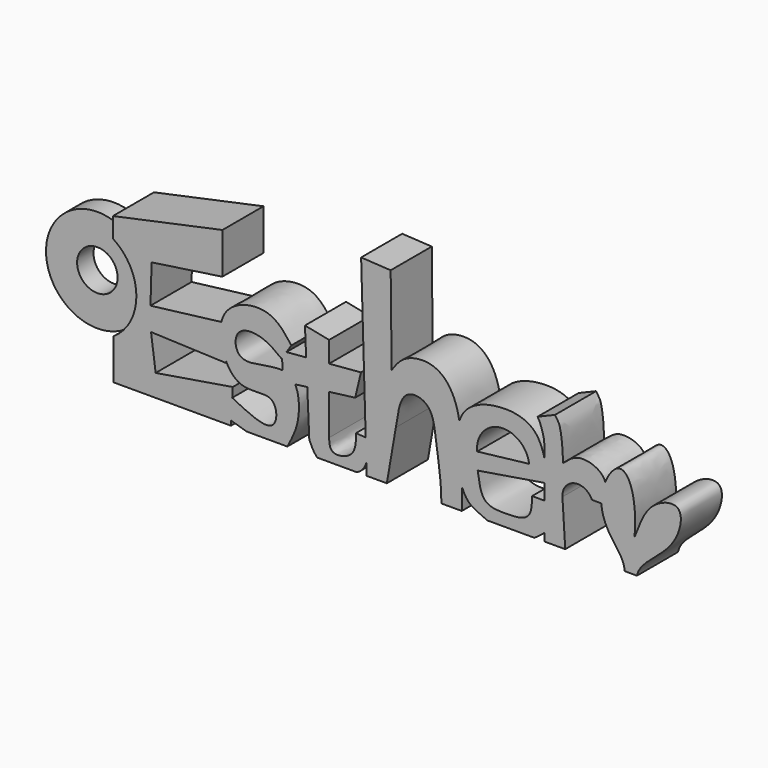
from build123d import *

# Parameters (mm, degrees)
F1_DEPTH = 5
F2_START = 1.5
F2_DEPTH = 2


# Not quite as in the source:
# - a feature names something its author has since deleted; it is built from what else it names


with BuildPart() as f1:
    # F0 (on Front) → F1 (new body)
    with BuildSketch(Plane.XZ):
        with BuildLine():
            Line((-14.6383177999, 11.432787973), (-25.3042323707, 9.1610242137))
            Line((-25.3042323707, 9.1610242137), (-25.2940563938, 7.2257657942))
            ThreePointArc((-25.2940563938, 7.2257657942), (-23.6221339238, 5.4180260022), (-23.0158091336, 3.0314765788))
            ThreePointArc((-23.0158091336, 3.0314765788), (-23.60964588, 0.6680626534), (-25.2500992867, -1.1339584576))
            Line((-25.2500992867, -1.1339584576), (-25.2293782792, -5.0746615769))
            Line((-25.2293782792, -5.0746615769), (-15.492977577, -5.0746615769))
            Line((-15.492977577, -5.0746615769), (-13.9721783602, -2.4893034869))
            add(Edge.make_bspline(
                [(-13.6837295023, -2.6371658395), (-13.7797644726, -2.5880426267), (-13.8759714164, -2.5386730568), (-13.9721783602, -2.4893034869)],
                knots=[0.9902207263, 0.9902207263, 0.9902207263, 0.9902207263, 1, 1, 1, 1], degree=3))
            Line((-13.6837295023, -2.6371658395), (-13.63845427, -1.7014753337))
            Line((-13.63845427, -1.7014753337), (-21.1411339112, -2.9332586315))
            Line((-21.1411339112, -2.9332586315), (-21.5890550329, 0.4261498349))
            Line((-21.5890550329, 0.4261498349), (-14.3103359526, 0.1461990572))
            Line((-14.3103359526, 0.1461990572), (-14.3137004114, 0.3514294783))
            add(Edge.make_bspline(
                [(-14.7392719458, 3.5156966528), (-14.9673627085, 2.527258961), (-14.7748693898, 1.3122008631), (-14.3137004114, 0.3514294783)],
                knots=[0.3602065009, 0.3602065009, 0.3602065009, 0.3602065009, 0.4667919333, 0.4667919333, 0.4667919333, 0.4667919333], degree=3))
            Line((-14.7392719458, 3.5156966528), (-21.6450438952, 2.6657553903))
            Line((-21.6450438952, 2.6657553903), (-21.5330644667, 6.4170949979))
            Line((-21.5330644667, 6.4170949979), (-14.6462776459, 7.4249175218))
            Line((-14.6462776459, 7.4249175218), (-14.6383177999, 11.432787973))
        make_face()
        with BuildLine():
            Line((-13.9721783602, -2.4893034869), (-15.492977577, -5.0746615769))
            Line((-15.492977577, -5.0746615769), (-13.8016725453, -5.0746615769))
            Line((-13.8016725453, -5.0746615769), (-13.780067623, -4.6281587181))
            Line((-13.780067623, -4.6281587181), (-13.6837295023, -2.6371658395))
            add(Edge.make_bspline(
                [(-13.6837295023, -2.6371658395), (-13.7797644726, -2.5880426267), (-13.8759714164, -2.5386730568), (-13.9721783602, -2.4893034869)],
                knots=[0.9902207263, 0.9902207263, 0.9902207263, 0.9902207263, 1, 1, 1, 1], degree=3))
        make_face()
        with BuildLine():
            add(Edge.make_bspline(
                [(-7.9252432167, 3.7256022903), (-8.6017964799, 4.6235767573), (-10.0658100387, 6.5667301891), (-14.0793719479, 5.5299447464), (-14.6901886794, 3.7284003591), (-14.7392719458, 3.5156966528)],
                knots=[0, 0, 0, 0, 0.1558600634, 0.3372701877, 0.3602065009, 0.3602065009, 0.3602065009, 0.3602065009], degree=3))
            Line((-14.7392719458, 3.5156966528), (-14.3663265189, 3.5615976338))
            Line((-14.3663265189, 3.5615976338), (-14.3137004114, 0.3514294783))
            add(Edge.make_bspline(
                [(-14.3137004114, 0.3514294783), (-14.0058860681, -0.2898521921), (-12.6382698651, -1.9789125391), (-9.3444686191, -0.5351869492), (-9.1851227698, -4.8542123742), (-11.9991293518, -3.498862068), (-13.6837295023, -2.6371658395)],
                knots=[0.4667919333, 0.4667919333, 0.4667919333, 0.4667919333, 0.537934023, 0.6943763321, 0.8186773195, 0.9902207263, 0.9902207263, 0.9902207263, 0.9902207263], degree=3))
            Line((-13.6837295023, -2.6371658395), (-13.780067623, -4.6281587181))
            Line((-13.780067623, -4.6281587181), (-12.2924484313, -5.0746615769))
            Line((-12.2924484313, -5.0746615769), (-8.3171737722, -5.0746615769))
            add(Edge.make_bspline(
                [(-7.5643111566, 0.5088960617), (-7.1593374225, -0.2359643215), (-7.0799460802, -2.8326585676), (-7.8565861691, -4.1742172582), (-8.3171737722, -5.0746615769)],
                knots=[0.6981935266, 0.6981935266, 0.6981935266, 0.6981935266, 0.8300505255, 1, 1, 1, 1], degree=3))
            Line((-7.5643111566, 0.5088960617), (-8.710907974, 0.3613812428))
            Line((-8.710907974, 0.3613812428), (-8.7705105138, 1.3070137316))
            add(Edge.make_bspline(
                [(-8.8770751744, 2.2698584316), (-9.5470148943, 2.7802809588), (-10.8445161237, 3.7606292374), (-13.6185783527, 3.5768971664), (-13.2844744483, 0.056692059), (-10.007786194, 1.4295023021), (-8.7705105138, 1.3070137316)],
                knots=[0, 0, 0, 0, 0.155258307, 0.2980121225, 0.4366297804, 0.6172059837, 0.6172059837, 0.6172059837, 0.6172059837], degree=3))
            Line((-8.8770751744, 2.2698584316), (-8.8352315589, 2.3338545874))
            Line((-8.8352315589, 2.3338545874), (-8.8770751744, 2.997730361))
            Line((-8.8770751744, 2.997730361), (-8.4011591955, 2.997730361))
            Line((-8.4011591955, 2.997730361), (-7.9252432167, 3.7256022903))
        make_face()
        Polygon((-8.8352315589, 2.3338545874), (-8.4011591955, 2.997730361), (-8.8770751744, 2.997730361), align=None)
        with BuildLine():
            Line((-8.710907974, 0.3613812428), (-7.5643111566, 0.5088960617))
            add(Edge.make_bspline(
                [(-8.7705105138, 1.3070137316), (-8.5861001566, 1.2887573629), (-8.0723941534, 1.1737189258), (-7.7303875658, 0.8143572001), (-7.5643111566, 0.5088960617)],
                knots=[0.6172059837, 0.6172059837, 0.6172059837, 0.6172059837, 0.644120052, 0.6981935266, 0.6981935266, 0.6981935266, 0.6981935266], degree=3))
            Line((-8.7705105138, 1.3070137316), (-8.710907974, 0.3613812428))
        make_face()
        with BuildLine():
            Line((-6.4865529854, 3.1603610324), (-8.4011591955, 2.997730361))
            Line((-8.4011591955, 2.997730361), (-8.8352315589, 2.3338545874))
            Line((-8.8352315589, 2.3338545874), (-8.7705105138, 1.3070137316))
            add(Edge.make_bspline(
                [(-8.7705105138, 1.3070137316), (-8.5861001566, 1.2887573629), (-8.0723941534, 1.1737189258), (-7.7303875658, 0.8143572001), (-7.5643111566, 0.5088960617)],
                knots=[0.6172059837, 0.6172059837, 0.6172059837, 0.6172059837, 0.644120052, 0.6981935266, 0.6981935266, 0.6981935266, 0.6981935266], degree=3))
            Line((-7.5643111566, 0.5088960617), (-6.3768543613, 0.6616676998))
            Line((-6.3768543613, 0.6616676998), (-6.4865529854, 3.1603610324))
        make_face()
        Polygon((-4.2509881896, 3.3502546), (-6.4865529854, 3.1603610324), (-6.3768543613, 0.6616676998), (-4.2509881896, 0.9351699096), align=None)
        Polygon((-6.6050835923, 5.8602275043), (-6.4865529854, 3.1603610324), (-4.2509881896, 3.3502546), (-4.2509881896, 5.389408509), align=None)
        Polygon((-1.1504360373, 3.6136220099), (-4.2509881896, 3.3502546), (-4.2509881896, 0.9351699096), (-1.7103374395, 1.2620360142), align=None)
        with BuildLine():
            add(Edge.make_bspline(
                [(-6.1813468373, -3.7915636042), (-5.9647248658, -4.2720436623), (-5.7481028943, -4.7525237205), (-5.3971613001, -5.0746615769)],
                knots=[0, 0, 0, 0, 0.1630961423, 0.1630961423, 0.1630961423, 0.1630961423], degree=3))
            Line((-5.3971613001, -5.0746615769), (-1.5808742849, -5.0746615769))
            add(Edge.make_bspline(
                [(-1.5808742849, -5.0746615769), (-1.2938921751, -4.9510178692), (-0.9318345489, -4.683797374), (-0.6953384614, -4.1697392882), (-0.6272426026, -3.9793869827)],
                knots=[0.5555288343, 0.5555288343, 0.5555288343, 0.5555288343, 0.6646108219, 0.7218728745, 0.7218728745, 0.7218728745, 0.7218728745], degree=3))
            Line((-0.6272426026, -3.9793869827), (-0.6898374488, -1.8284651253))
            Line((-0.6898374488, -1.8284651253), (-1.6263508447, -1.7401147499))
            add(Edge.make_bspline(
                [(-4.2509881896, -2.9911710565), (-4.2323081287, -3.4463528642), (-4.1905224115, -4.4645560932), (-1.6583641706, -3.9931371174), (-1.6372868286, -2.5097635024), (-1.6263508447, -1.7401147499)],
                knots=[0, 0, 0, 0, 0.2800532554, 0.6264554606, 1, 1, 1, 1], degree=3))
            Line((-4.2509881896, -2.9911710565), (-4.2509881896, 0.9351699096))
            Line((-4.2509881896, 0.9351699096), (-6.3768543613, 0.6616676998))
            Line((-6.3768543613, 0.6616676998), (-6.1813468373, -3.7915636042))
        make_face()
        with BuildLine():
            Line((-0.6898374488, -1.8284651253), (-0.6272426026, -3.9793869827))
            add(Edge.make_bspline(
                [(-0.6272426026, -3.9793869827), (-0.4222294069, -3.4063017004), (-0.286190737, -2.2858872911), (-0.3532046371, -1.975727647), (-0.3786801556, -1.8578196052)],
                knots=[0.7218728745, 0.7218728745, 0.7218728745, 0.7218728745, 0.8942692082, 1, 1, 1, 1], degree=3))
            Line((-0.3786801556, -1.8578196052), (-0.6898374488, -1.8284651253))
        make_face()
        with BuildLine():
            add(Edge.make_bspline(
                [(-0.6272426026, -3.9793869827), (-0.4222294069, -3.4063017004), (-0.286190737, -2.2858872911), (-0.3532046371, -1.975727647), (-0.3786801556, -1.8578196052)],
                knots=[0.7218728745, 0.7218728745, 0.7218728745, 0.7218728745, 0.8942692082, 1, 1, 1, 1], degree=3))
            Line((-0.6272426026, -3.9793869827), (-0.5953685741, -5.0746615769))
            Line((-0.5953685741, -5.0746615769), (1.3691666113, -5.0746615769))
            Line((1.3691666113, -5.0746615769), (2.2456591552, 0))
            add(Edge.make_bspline(
                [(2.2456591552, 0), (2.3908026267, 0.7936117461), (2.5869429568, 3.7215165763), (5.8742621, 3.2511142124), (6.1260228489, -0.407677054), (6.6578289119, -2.7761030612), (6.6858463929, -5.0746615769)],
                knots=[0, 0, 0, 0, 0.2471109773, 0.4464517653, 0.6875591648, 1, 1, 1, 1], degree=3))
            Line((6.6858463929, -5.0746615769), (8.663286429, -5.0746615769))
            add(Edge.make_bspline(
                [(8.710870771, -3.0764876678), (8.6993593613, -3.7320763082), (8.6815142362, -4.4006243358), (8.663286429, -5.0746615769)],
                knots=[0.9262146344, 0.9262146344, 0.9262146344, 0.9262146344, 1, 1, 1, 1], degree=3))
            add(Edge.make_bspline(
                [(8.0512207127, -0.910654593), (8.252229366, -1.6640447479), (8.4422246003, -2.4385569534), (8.7108707672, -3.0764876686)],
                knots=[0, 0, 0, 0, 0.3507878296, 0.3507878296, 0.3507878296, 0.3507878296], degree=3))
            add(Edge.make_bspline(
                [(8.4317405273, 2.5746243527), (8.0849358238, 1.5628637249), (8.0694106027, 0.2953210601), (8.0512207127, -0.910654593)],
                knots=[0.7991343328, 0.7991343328, 0.7991343328, 0.7991343328, 1, 1, 1, 1], degree=3))
            add(Edge.make_bspline(
                [(1.8364099315, 4.7862562304), (2.210613761, 5.3249179502), (3.0152292151, 6.4814511219), (6.1941571435, 6.8876174891), (7.87519526, 4.9466794186), (8.3455981531, 3.049626497), (8.4317405273, 2.5746243527)],
                knots=[0, 0, 0, 0, 0.177954814, 0.3863462091, 0.6194415241, 0.6900838123, 0.6900838123, 0.6900838123, 0.6900838123], degree=3))
            Line((1.8364099315, 4.7862562304), (1.7422460899, 13.3080812389))
            Line((1.7422460899, 13.3080812389), (-1.1350971628, 13.471817734))
            Line((-1.1350971628, 13.471817734), (-0.6898374488, -1.8284651253))
            Line((-0.6898374488, -1.8284651253), (-0.3786801556, -1.8578196052))
        make_face()
        with BuildLine():
            add(Edge.make_bspline(
                [(8.0512207127, -0.910654593), (8.252229366, -1.6640447479), (8.4422246003, -2.4385569534), (8.7108707672, -3.0764876686)],
                knots=[0, 0, 0, 0, 0.3507878296, 0.3507878296, 0.3507878296, 0.3507878296], degree=3))
            add(Edge.make_bspline(
                [(8.4317405273, 2.5746243527), (8.7196823558, 0.9868693469), (8.7477100358, -0.9784471769), (8.710870771, -3.0764876678)],
                knots=[0.6900838123, 0.6900838123, 0.6900838123, 0.6900838123, 0.9262146344, 0.9262146344, 0.9262146344, 0.9262146344], degree=3))
            add(Edge.make_bspline(
                [(8.4317405273, 2.5746243527), (8.0849358238, 1.5628637249), (8.0694106027, 0.2953210601), (8.0512207127, -0.910654593)],
                knots=[0.7991343328, 0.7991343328, 0.7991343328, 0.7991343328, 1, 1, 1, 1], degree=3))
        make_face()
        with BuildLine():
            add(Edge.make_bspline(
                [(8.7108707672, -3.0764876686), (8.8667237067, -3.4465781049), (9.4483604115, -4.4805677283), (10.477562838, -4.733368314), (11.1586264227, -5.0746615769)],
                knots=[0.3507878296, 0.3507878296, 0.3507878296, 0.3507878296, 0.5542946021, 1, 1, 1, 1], degree=3))
            Line((11.1586264227, -5.0746615769), (15.7429713916, -5.0746615769))
            add(Edge.make_bspline(
                [(16.7163866144, -4.3206934491), (16.4451170047, -4.58215224), (16.0905474083, -4.8029155356), (15.7429713916, -5.0746615769)],
                knots=[0.6955604726, 0.6955604726, 0.6955604726, 0.6955604726, 1, 1, 1, 1], degree=3))
            Line((16.7163866144, -4.3206934491), (16.7163866144, -1.5704254551))
            Line((16.7163866144, -1.5704254551), (15.5099269965, -1.5704254551))
            add(Edge.make_bspline(
                [(10.216508766, -1.1043384754), (10.3478194791, -2.054062847), (10.5991695735, -3.8719899981), (12.990667886, -3.9301543375), (15.4561978016, -3.8120714775), (15.4923194324, -2.3050340044), (15.5099269965, -1.5704254551)],
                knots=[0, 0, 0, 0, 0.269202223, 0.5152969062, 0.7637304692, 1, 1, 1, 1], degree=3))
            Line((10.216508766, -1.1043384754), (16.7163866144, -0.0474281658))
            Line((16.7163866144, -0.0474281658), (16.7163866144, 2.0553055108))
            add(Edge.make_bspline(
                [(16.7163866144, 2.0553055108), (16.539898754, 2.7887249895), (15.7518134558, 4.7816758833), (12.2003044072, 5.3803861966), (9.2138809368, 4.2930120801), (8.5376393761, 2.8835713904), (8.4317405273, 2.5746243527)],
                knots=[0.1245888859, 0.1245888859, 0.1245888859, 0.1245888859, 0.2547857387, 0.4959089273, 0.737798824, 0.7991343328, 0.7991343328, 0.7991343328, 0.7991343328], degree=3))
            add(Edge.make_bspline(
                [(8.4317405273, 2.5746243527), (8.7196823558, 0.9868693469), (8.7477100358, -0.9784471769), (8.710870771, -3.0764876678)],
                knots=[0.6900838123, 0.6900838123, 0.6900838123, 0.6900838123, 0.9262146344, 0.9262146344, 0.9262146344, 0.9262146344], degree=3))
        make_face()
        with BuildLine():
            ThreePointArc((10.1624862787, 0.5105888854), (12.4033566317, 3.2969815496), (15.2237921826, 1.0991127361))
            Line((15.2237921826, 1.0991127361), (10.1624862787, 0.5105888854))
        make_face(mode=Mode.SUBTRACT)
        with BuildLine():
            add(Edge.make_bspline(
                [(17.0080644244, 0), (16.9627338224, 0.6199401127), (16.885272616, 1.3534765972), (16.7163866144, 2.0553055108)],
                knots=[0, 0, 0, 0, 0.1245888859, 0.1245888859, 0.1245888859, 0.1245888859], degree=3))
            Line((16.7163866144, 2.0553055108), (16.7163866144, -0.0474281658))
            Line((16.7163866144, -0.0474281658), (17.0080644244, 0))
        make_face()
        with BuildLine():
            Line((16.7163866144, -1.5704254551), (16.7163866144, -4.3206934491))
            add(Edge.make_bspline(
                [(17.0746485373, -1.5704254551), (17.2000978678, -2.4016480145), (17.3809146938, -3.5273932374), (16.8663492206, -4.1761544358), (16.7163866144, -4.3206934491)],
                knots=[0, 0, 0, 0, 0.527260953, 0.6955604726, 0.6955604726, 0.6955604726, 0.6955604726], degree=3))
            Line((17.0746485373, -1.5704254551), (16.7163866144, -1.5704254551))
        make_face()
        with BuildLine():
            Line((16.7163866144, 3.1534400123), (16.7163866144, 2.0553055108))
            add(Edge.make_bspline(
                [(17.0080644244, 0), (16.9627338224, 0.6199401127), (16.885272616, 1.3534765972), (16.7163866144, 2.0553055108)],
                knots=[0, 0, 0, 0, 0.1245888859, 0.1245888859, 0.1245888859, 0.1245888859], degree=3))
            Line((17.0080644244, 0), (16.7163866144, -0.0474281658))
            Line((16.7163866144, -0.0474281658), (16.7163866144, -1.5704254551))
            Line((16.7163866144, -1.5704254551), (17.0746485373, -1.5704254551))
            add(Edge.make_bspline(
                [(17.0746485373, -1.5704254551), (17.2000978678, -2.4016480145), (17.3809146938, -3.5273932374), (16.8663492206, -4.1761544358), (16.7163866144, -4.3206934491)],
                knots=[0, 0, 0, 0, 0.527260953, 0.6955604726, 0.6955604726, 0.6955604726, 0.6955604726], degree=3))
            Line((16.7163866144, -4.3206934491), (16.7163866144, -5.0746615769))
            Line((16.7163866144, -5.0746615769), (18.7378928823, -5.0746615769))
            Line((18.7378928823, -5.0746615769), (18.4655259078, -0.6776052563))
            ThreePointArc((18.4655259078, -0.6776052563), (19.6137552416, 0.8696064789), (21.3330804954, 0))
            Line((21.3330804954, 0), (22.2573663261, 0))
            add(Edge.make_bspline(
                [(22.2573663261, 0), (22.2435884919, 0.2629694157), (22.2721798746, 0.916034239), (22.4760388023, 1.5992350752), (22.6331089349, 1.9708111909)],
                knots=[0.3663867783, 0.3663867783, 0.3663867783, 0.3663867783, 0.4147064149, 0.4837509131, 0.4837509131, 0.4837509131, 0.4837509131], degree=3))
            add(Edge.make_bspline(
                [(18.5343598641, 2.2593869314), (19.0343468508, 2.6551000146), (19.9223877685, 3.5486369075), (22.0734764179, 2.9796106894), (22.5633467803, 2.1343263315), (22.6331089349, 1.9708111909)],
                knots=[0, 0, 0, 0, 0.3000824589, 0.6466861365, 0.7228510598, 0.7228510598, 0.7228510598, 0.7228510598], degree=3))
            add(Edge.make_bspline(
                [(17.7444275279, 6.1163512452), (17.9296281498, 5.8005482522), (18.3026359953, 5.5017776291), (18.5093903106, 3.4111286387), (18.5343598641, 2.2593869314)],
                knots=[0, 0, 0, 0, 0.3403899819, 1, 1, 1, 1], degree=3))
            Line((17.7444275279, 6.1163512452), (16.0494788038, 5.4101223262))
            add(Edge.make_bspline(
                [(16.0494788038, 5.4101223262), (16.203733589, 5.1583820337), (16.4265981269, 4.634740352), (16.6893511914, 3.7935902225), (16.7163866144, 3.1534400123)],
                knots=[0, 0, 0, 0, 0.4235101645, 1, 1, 1, 1], degree=3))
        make_face()
        with BuildLine():
            add(Edge.make_bspline(
                [(24.5242888786, -5.0746615769), (24.4924619967, -4.0880189994), (23.0751204927, -2.7440868169), (22.3047264604, -0.9039350225), (22.2573663261, 0)],
                knots=[0, 0, 0, 0, 0.2002921331, 0.3663867783, 0.3663867783, 0.3663867783, 0.3663867783], degree=3))
            Line((24.5242888786, -5.0746615769), (25.7187202118, -5.0746615769))
            add(Edge.make_bspline(
                [(25.4927472689, -1.8247166888), (26.0370331286, -0.4673113977), (26.7235093439, 1.6761399963), (30.5561848801, 2.8142060101), (29.5562406084, -2.067748533), (25.9773616035, -3.7167908573), (25.7187202118, -5.0746615769)],
                knots=[0, 0, 0, 0, 0.2575446618, 0.4617515065, 0.704906762, 1, 1, 1, 1], degree=3))
            add(Edge.make_bspline(
                [(22.6331089349, 1.9708111909), (22.9425524074, 2.7028523605), (23.7969116037, 3.8598153004), (25.2634960825, 3.1203083475), (25.6630058048, 0.3790322021), (25.4927472689, -1.8247166888)],
                knots=[0.4837509131, 0.4837509131, 0.4837509131, 0.4837509131, 0.6197753053, 0.7399541503, 1, 1, 1, 1], degree=3))
            add(Edge.make_bspline(
                [(22.6331089349, 1.9708111909), (22.8869594788, 1.3758122605), (22.8959645087, 0.6321071961), (22.970518717, 0)],
                knots=[0.7228510598, 0.7228510598, 0.7228510598, 0.7228510598, 1, 1, 1, 1], degree=3))
            Line((22.970518717, 0), (22.2573663261, 0))
        make_face()
        with BuildLine():
            add(Edge.make_bspline(
                [(22.2573663261, 0), (22.2435884919, 0.2629694157), (22.2721798746, 0.916034239), (22.4760388023, 1.5992350752), (22.6331089349, 1.9708111909)],
                knots=[0.3663867783, 0.3663867783, 0.3663867783, 0.3663867783, 0.4147064149, 0.4837509131, 0.4837509131, 0.4837509131, 0.4837509131], degree=3))
            Line((22.2573663261, 0), (22.970518717, 0))
            add(Edge.make_bspline(
                [(22.6331089349, 1.9708111909), (22.8869594788, 1.3758122605), (22.8959645087, 0.6321071961), (22.970518717, 0)],
                knots=[0.7228510598, 0.7228510598, 0.7228510598, 0.7228510598, 1, 1, 1, 1], degree=3))
        make_face()
        with BuildLine():
            Line((-14.3663265189, 3.5615976338), (-14.7392719458, 3.5156966528))
            add(Edge.make_bspline(
                [(-14.7392719458, 3.5156966528), (-14.9673627085, 2.527258961), (-14.7748693898, 1.3122008631), (-14.3137004114, 0.3514294783)],
                knots=[0.3602065009, 0.3602065009, 0.3602065009, 0.3602065009, 0.4667919333, 0.4667919333, 0.4667919333, 0.4667919333], degree=3))
            Line((-14.3137004114, 0.3514294783), (-14.3663265189, 3.5615976338))
        make_face()
    extrude(amount=F1_DEPTH)

    # F0 (on Front) → F2 (join)
    with BuildSketch(Plane.XZ.offset(F2_START)):
        with BuildLine():
            Line((-25.2879420917, 6.0629531576), (-25.2940563938, 7.2257657942))
            ThreePointArc((-25.2940563938, 7.2257657942), (-33.0157400134, 3.0051859392), (-25.2500992867, -1.1339584576))
            Line((-25.2500992867, -1.1339584576), (-25.2563075848, 0.0467302614))
            Line((-25.2563075848, 0.0467302614), (-25.2879420917, 6.0629531576))
        make_face()
        with BuildLine():
            Line((-27.2635575384, 6.0629531576), (-25.2879420917, 6.0629531576))
            Line((-25.2879420917, 6.0629531576), (-25.2879420917, 0))
            Line((-25.2879420917, 0), (-27.2635575384, 0))
            Line((-27.2635575384, 0), (-27.2635575384, 1.21003361))
            ThreePointArc((-27.2635575384, 1.21003361), (-29.9864782969, 3.0314765788), (-27.2635575384, 4.8529195476))
            Line((-27.2635575384, 4.8529195476), (-27.2635575384, 6.0629531576))
        make_face(mode=Mode.SUBTRACT)
        with BuildLine():
            Line((-25.2879420917, 0), (-25.2879420917, 6.0629531576))
            Line((-25.2879420917, 6.0629531576), (-27.2635575384, 6.0629531576))
            Line((-27.2635575384, 6.0629531576), (-27.2635575384, 4.8529195476))
            ThreePointArc((-27.2635575384, 4.8529195476), (-26.3778262319, 4.1271722321), (-26.0451399704, 3.0314765788))
            ThreePointArc((-26.0451399704, 3.0314765788), (-26.3778262319, 1.9357809255), (-27.2635575384, 1.21003361))
            Line((-27.2635575384, 1.21003361), (-27.2635575384, 0))
            Line((-27.2635575384, 0), (-25.2879420917, 0))
        make_face()
        with BuildLine():
            ThreePointArc((-23.0158091336, 3.0314765788), (-23.6221339238, 5.4180260022), (-25.2940563938, 7.2257657942))
            Line((-25.2940563938, 7.2257657942), (-25.2879420917, 6.0629531576))
            Line((-25.2879420917, 6.0629531576), (-25.2563075848, 0.0467302614))
            Line((-25.2563075848, 0.0467302614), (-25.2500992867, -1.1339584576))
            ThreePointArc((-25.2500992867, -1.1339584576), (-23.60964588, 0.6680626534), (-23.0158091336, 3.0314765788))
        make_face()
    extrude(amount=F2_DEPTH)


solid = f1.part
